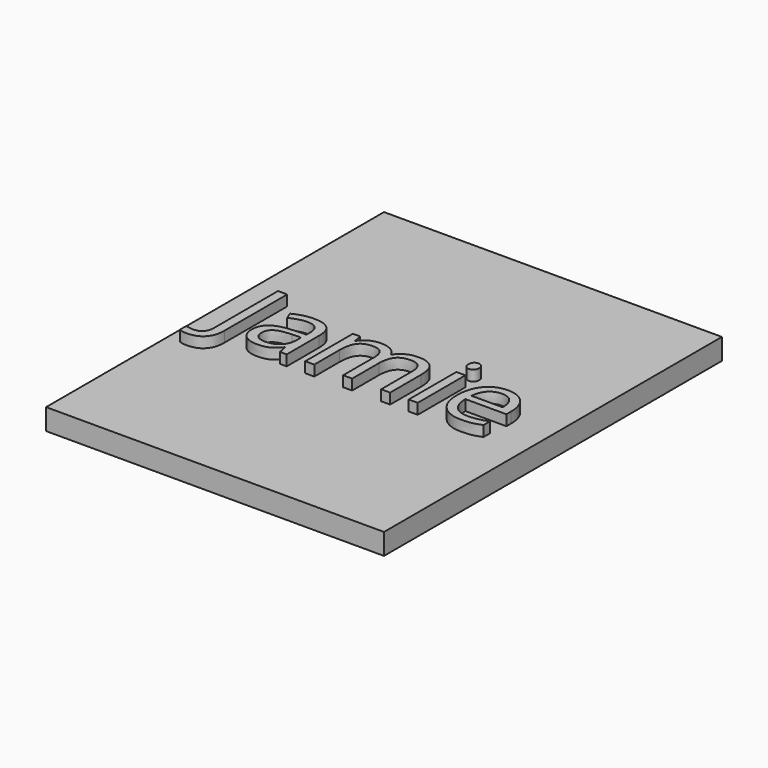
from build123d import *

# Parameters (mm, degrees)
F0_W         = 101.6
F0_H         = 127
F1_DEPTH     = 6.35
F2_TEXT_SIZE = 33.4465933808
F3_DEPTH     = 3.175


# Not quite as in the source:
# - a length typed as a fraction of an inch, garbled in the dataset ("3 / 203.2 mm" for 3/8 in), is restored
# - Text() gives the source's letters only with a copy of the font that has no kerning and outlines rounded to 1/6400 em; it was checked with that copy


with BuildPart() as f1:
    # F0 (on Top) → F1 (new body)
    with BuildSketch(Plane.XY):
        Rectangle(F0_W, F0_H)
    extrude(amount=F1_DEPTH)

    # F2 (on face) → F3 (join)
    with BuildSketch(Plane.XY.offset(6.35)):
        with Locations((-44.45, -12.0407736171)):
            Text('Jamie', F2_TEXT_SIZE, font='Open Sans', text_align=(TextAlign.LEFT, TextAlign.BOTTOM))
    extrude(amount=F3_DEPTH)


solid = f1.part
